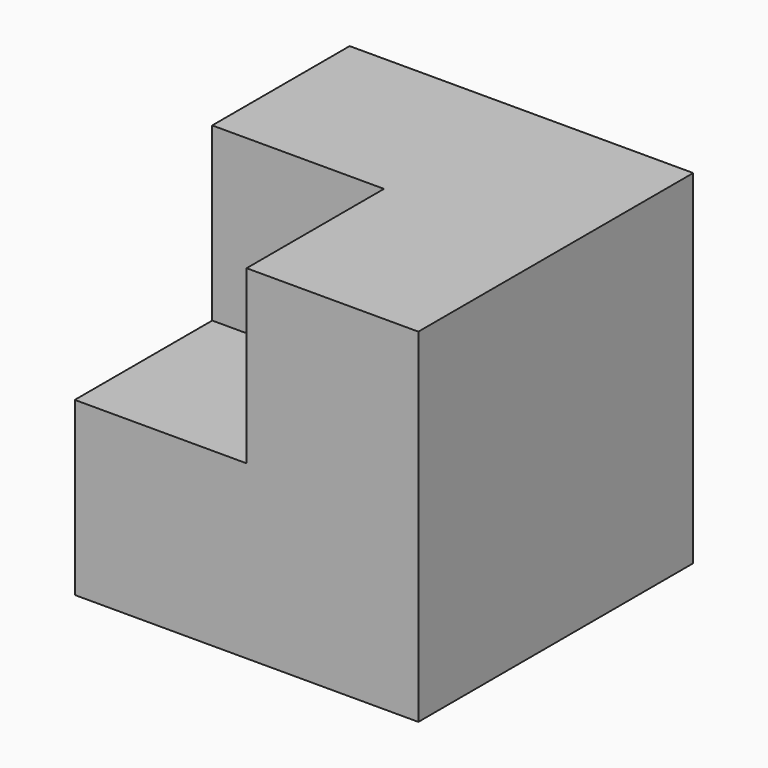
from build123d import *

# Parameters (mm, degrees)
F0_W     = 50.8
F0_H     = 50.8
F1_DEPTH = 50.8
F2_W     = 25.4
F2_H     = 25.4
F3_DEPTH = 25.4


# Not quite as in the source:
# - a feature names something its author has since deleted; it is built from what else it names


with BuildPart() as f1:
    # F0 (on Front) → F1 (new body)
    with BuildSketch(Plane.XZ):
        with Locations((-25.4, 25.4)):
            Rectangle(F0_W, F0_H)
    extrude(amount=F1_DEPTH)

    # F2 (on face) → F3 (cut)
    with BuildSketch(Plane.XZ.offset(50.8)):
        with Locations((-38.1, 38.1)):
            Rectangle(F2_W, F2_H)
    extrude(amount=-F3_DEPTH, mode=Mode.SUBTRACT)


solid = f1.part
